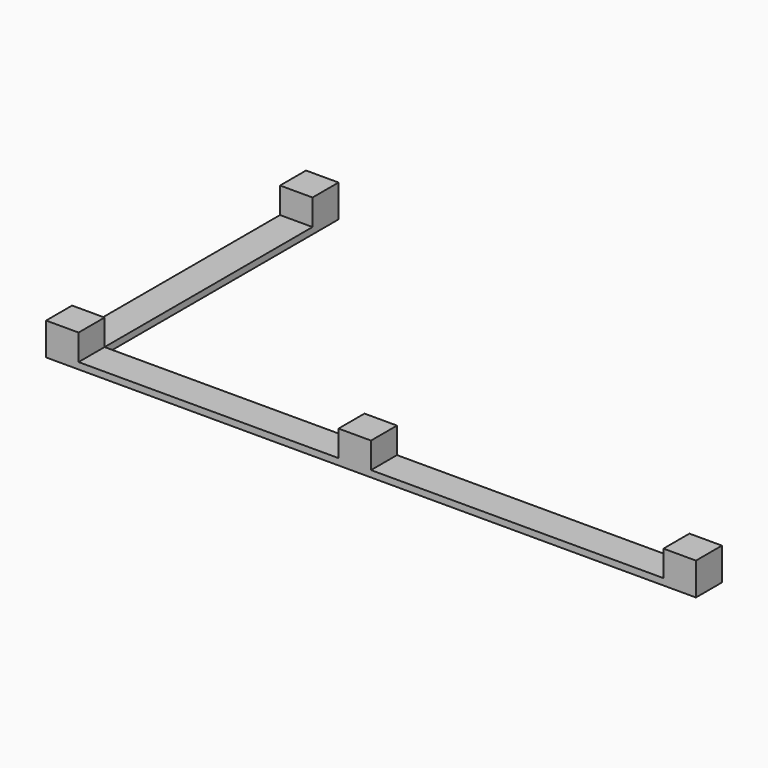
from build123d import *

# Parameters (mm, degrees)
F0_W     = 5
F0_H     = 5
F1_DEPTH = 5
F0_W_2   = 45
F0_W_3   = 40
F0_H_2   = 40
F2_DEPTH = 1


# Not quite as in the source:
# - a feature of the source that left no trace in its solid (it failed there, or was rolled back) is left out


with BuildPart() as f1:
    # F0 (on Top) → F1 (new body)
    with BuildSketch(Plane.XY):
        with Locations((-47.5, 45)):
            Rectangle(F0_W, F0_H)
    extrude(amount=F1_DEPTH)



with BuildPart() as f1b:
    # F0 (on Top) → F1, piece 2 (new body)
    with BuildSketch(Plane.XY):
        with Locations((-47.5, 0)):
            Rectangle(F0_W, F0_H)
    extrude(amount=F1_DEPTH)


with BuildPart() as f1c:
    # F0 (on Top) → F1, piece 3 (new body)
    with BuildSketch(Plane.XY):
        with Locations((-2.5, 0)):
            Rectangle(F0_W, F0_H)
    extrude(amount=F1_DEPTH)


with BuildPart() as f1d:
    # F0 (on Top) → F1, piece 4 (new body)
    with BuildSketch(Plane.XY):
        with Locations((47.5, 0)):
            Rectangle(F0_W, F0_H)
    extrude(amount=F1_DEPTH)


with BuildPart() as f1_1:
    add(f1.part)

    add(f1b.part)  # F2 merges F1b

    add(f1c.part)  # F2 merges F1c

    add(f1d.part)  # F2 merges F1d
    # F0 (on Top) → F2 (join)
    with BuildSketch(Plane.XY):
        with Locations((47.5, 0)):
            Rectangle(F0_W, F0_H)
        with Locations((22.5, 0)):
            Rectangle(F0_W_2, F0_H)
        with Locations((-2.5, 0)):
            Rectangle(F0_W, F0_H)
        with Locations((-25, 0)):
            Rectangle(F0_W_3, F0_H)
        with Locations((-47.5, 0)):
            Rectangle(F0_W, F0_H)
        with Locations((-47.5, 22.5)):
            Rectangle(F0_W, F0_H_2)
        with Locations((-47.5, 45)):
            Rectangle(F0_W, F0_H)
    extrude(amount=F2_DEPTH)


solid = f1_1.part
